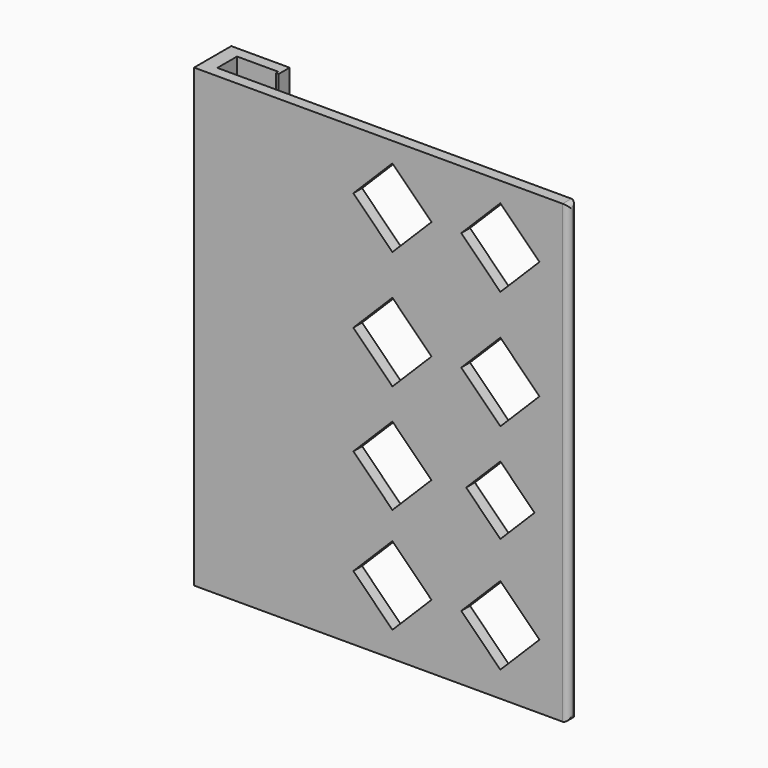
from build123d import *

# Parameters (mm, degrees)
F0_W     = 197.0480888034
F0_H     = 6
F0_W_2   = 7.9519111966
F0_H_2   = 13.5
F0_W_3   = 1.5
F0_H_3   = 1.5
F1_DEPTH = 250
F3_DEPTH = 25
F4_R     = 2.99999


# Not quite as in the source:
# - a fillet or chamfer is up to 0.001 mm smaller than in the source, because OpenCascade refuses the exact size


with BuildPart() as f1:
    # F0 (on Top) → F1 (new body)
    with BuildSketch(Plane.XY):
        with Locations((106.4759555983, 3)):
            Rectangle(F0_W, F0_H)
        with Locations((3.9759555983, 12.75)):
            Rectangle(F0_W_2, F0_H_2)
        with Locations((3.9759555983, 3)):
            Rectangle(F0_W_2, F0_H)
        with Locations((3.9759555983, 22.5)):
            Rectangle(F0_W_2, F0_H)
        Polygon((7.9519111966, 25.5), (7.9519111966, 19.5), (30.5, 19.5), (32, 19.5), (32, 25.5), align=None)
        with Locations((31.25, 18.75)):
            Rectangle(F0_W_3, F0_H_3)
    extrude(amount=F1_DEPTH)

    # F2 (on face) → F3 (cut)
    with BuildSketch(Plane.XZ):
        Polygon((87.3010246393, 35.425593216), (108.7266178553, 14), (130.1522110713, 35.425593216), (108.7266178553, 56.851186432), align=None)
        Polygon((146.474054042, 35.425593216), (167.8996472581, 14), (189.3252404741, 35.425593216), (167.8996472581, 56.851186432), align=None)
        Polygon((149.1576427927, 95.8152501475), (167.8996472581, 77.0732456821), (186.6416517235, 95.8152501475), (167.8996472581, 114.5572546129), align=None)
        Polygon((87.3569478805, 93.1875846381), (108.7266178553, 71.8179146634), (130.09628783, 93.1875846381), (108.7266178553, 114.5572546129), align=None)
        Polygon((87.3010246393, 152.8602018807), (108.7266178553, 131.4346086647), (130.1522110713, 152.8602018807), (108.7266178553, 174.2857950967), align=None)
        Polygon((146.474054042, 152.8602018807), (167.8996472581, 131.4346086647), (189.3252404741, 152.8602018807), (167.8996472581, 174.2857950967), align=None)
        Polygon((146.474054042, 217.7387669785), (167.8996472581, 196.3131737625), (189.3252404741, 217.7387669785), (167.8996472581, 239.1643601945), align=None)
        Polygon((87.3010246393, 217.7387669785), (108.7266178553, 196.3131737625), (130.1522110713, 217.7387669785), (108.7266178553, 239.1643601945), align=None)
    extrude(amount=-F3_DEPTH, mode=Mode.SUBTRACT)

    # F4 (radius 3 in the source; OpenCascade refuses exactly that, so slightly less here)
    f4_edges = [f1.edges().sort_by_distance(p)[0] for p in [
        (205, 0, 125),
        (205, 6, 125),
        (205, 3, 0),
        (205, 3, 250),
    ]]
    fillet(f4_edges, radius=F4_R)


solid = f1.part
